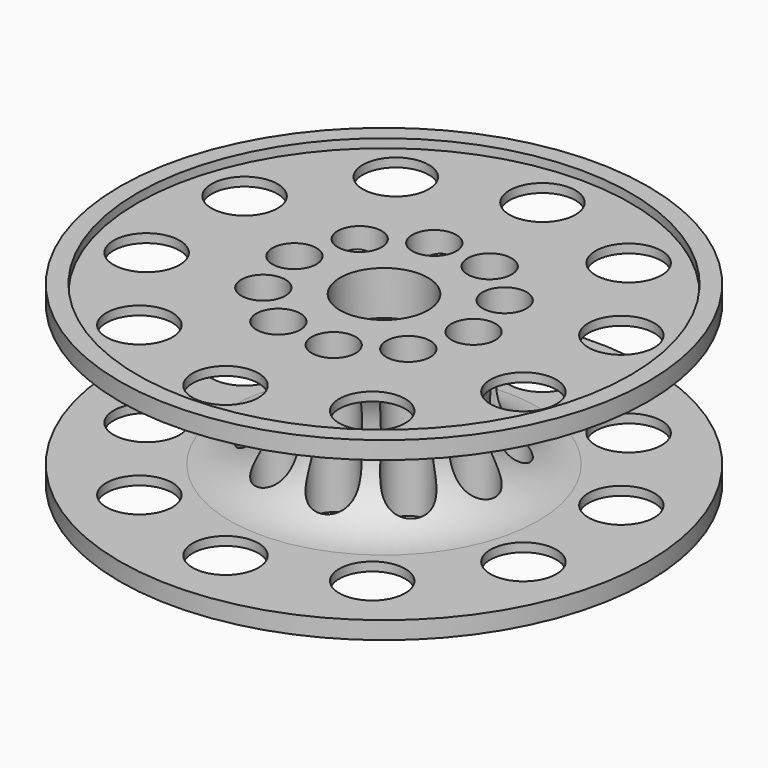
from build123d import *

# Parameters (mm, degrees)
F2_R     = 4.7625
F2_R_2   = 3.175
F3_DEPTH = 24.131
F4_R     = 6.35
F5_DEPTH = 6.35
F6_R     = 3.175
F7_DEPTH = 17.781


# Not quite as in the source:
# - a feature names something its author has since deleted; it is built from what else it names


with BuildPart() as f1:
    # F0 (on Front) → F1 (revolve)
    with BuildSketch(Plane.XZ):
        with BuildLine():
            Line((38.1, 22.86), (38.1, 25.4))
            Line((38.1, 25.4), (35.56, 25.4))
            Line((35.56, 25.4), (35.56, 24.13))
            Line((35.56, 24.13), (0, 24.13))
            Line((0, 24.13), (0, 1.27))
            Line((0, 1.27), (35.56, 1.27))
            Line((35.56, 1.27), (35.56, 0))
            Line((35.56, 0), (38.1, 0))
            Line((38.1, 0), (38.1, 2.54))
            Line((38.1, 2.54), (22.225, 2.54))
            ThreePointArc((22.225, 2.54), (15.4898079092, 5.3298079092), (12.7, 12.065))
            Line((12.7, 12.065), (12.7, 13.335))
            ThreePointArc((12.7, 13.335), (15.4898079092, 20.0701920908), (22.225, 22.86))
            Line((22.225, 22.86), (38.1, 22.86))
        make_face()
    revolve(axis=Axis((0, 0, 36.7639224648), (0, 0, 1)))

    # F2 (on face) → F3 (cut, through all)
    with BuildSketch(Plane.XY.offset(24.13)):
        with Locations((0, 28.575)):
            Circle(F2_R)
        with Locations((16.7959635843, 23.1176606143)):
            Circle(F2_R)
        with Locations((27.1764399531, 8.8301606143)):
            Circle(F2_R)
        with Locations((27.1764399531, -8.8301606143)):
            Circle(F2_R)
        with Locations((16.7959635843, -23.1176606143)):
            Circle(F2_R)
        with Locations((0, -28.575)):
            Circle(F2_R)
        with Locations((-16.7959635843, -23.1176606143)):
            Circle(F2_R)
        with Locations((-27.1764399531, -8.8301606143)):
            Circle(F2_R)
        with Locations((-27.1764399531, 8.8301606143)):
            Circle(F2_R)
        with Locations((-16.7959635843, 23.1176606143)):
            Circle(F2_R)
        with Locations((-3.3550663727, 13.2604649102)):
            Circle(F2_R_2)
        with Locations((-10.5086114255, 8.7558829313)):
            Circle(F2_R_2)
        with Locations((-13.6482240884, 0.9068512742)):
            Circle(F2_R_2)
        with Locations((-11.5746790355, -7.2885667469)):
            Circle(F2_R_2)
        with Locations((-5.08, -12.7)):
            Circle(F2_R_2)
        with Locations((3.3550663727, -13.2604649102)):
            Circle(F2_R_2)
        with Locations((10.5086114255, -8.7558829313)):
            Circle(F2_R_2)
        with Locations((13.6482240884, -0.9068512742)):
            Circle(F2_R_2)
        with Locations((11.5746790355, 7.2885667469)):
            Circle(F2_R_2)
        with Locations((5.08, 12.7)):
            Circle(F2_R_2)
    extrude(amount=-F3_DEPTH, mode=Mode.SUBTRACT)

    # F4 (on face) → F5 (cut)
    with BuildSketch(Plane.XY.offset(24.13)):
        Circle(F4_R)
    extrude(amount=-F5_DEPTH, mode=Mode.SUBTRACT)

    # F6 (on face) → F7 (cut, through all)
    with BuildSketch(Plane.XY.offset(17.78)):
        Circle(F6_R)
    extrude(amount=-F7_DEPTH, mode=Mode.SUBTRACT)


solid = f1.part
